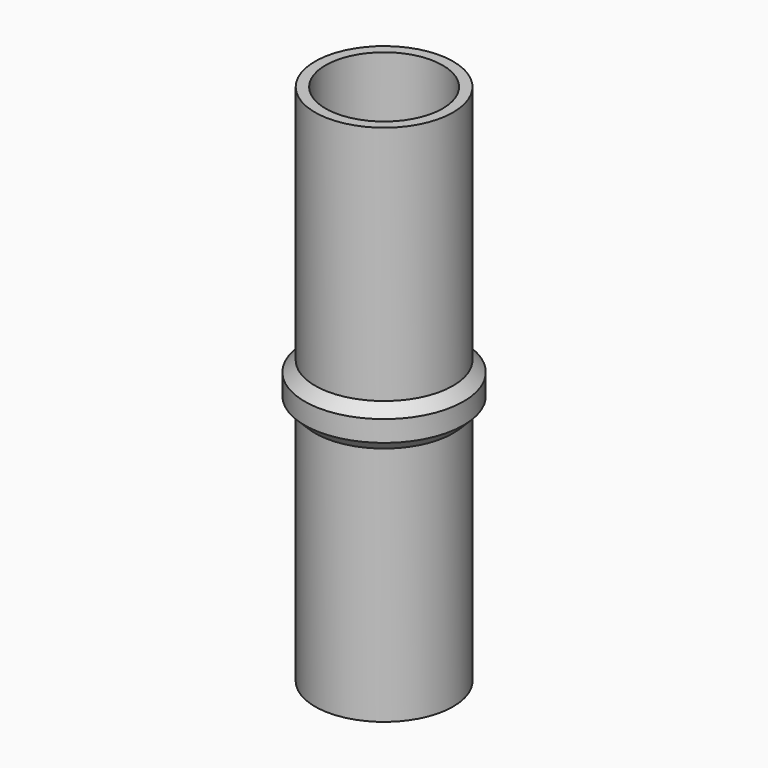
from build123d import *

# Parameters (mm, degrees)
F0_R     = 16.5
F0_R_2   = 14
F1_DEPTH = 125
F0_R_3   = 19
F2_DEPTH = 65
F3_DEPTH = 60
F4_SIZE  = 2.49999


# Not quite as in the source:
# - a fillet or chamfer is up to 0.001 mm smaller than in the source, because OpenCascade refuses the exact size


with BuildPart() as f1:
    # F0 (on Top) → F1 (new body)
    with BuildSketch(Plane.XY):
        Circle(F0_R)
        Circle(F0_R_2, mode=Mode.SUBTRACT)
    extrude(amount=F1_DEPTH)

    # F0 (on Top) → F2 (join)
    with BuildSketch(Plane.XY):
        Circle(F0_R_3)
        Circle(F0_R, mode=Mode.SUBTRACT)
    extrude(amount=F2_DEPTH)

    # F0 (on Top) → F3 (cut)
    with BuildSketch(Plane.XY):
        Circle(F0_R_3)
        Circle(F0_R, mode=Mode.SUBTRACT)
    extrude(amount=F3_DEPTH, mode=Mode.SUBTRACT)

    # F4 (size 2.5 in the source; OpenCascade refuses exactly that, so slightly less here)
    f4_edges = [f1.edges().sort_by_distance(p)[0] for p in [
        (-16.5, 0, 60),
        (-16.5, 0, 65),
    ]]
    chamfer(f4_edges, length=F4_SIZE)


solid = f1.part
